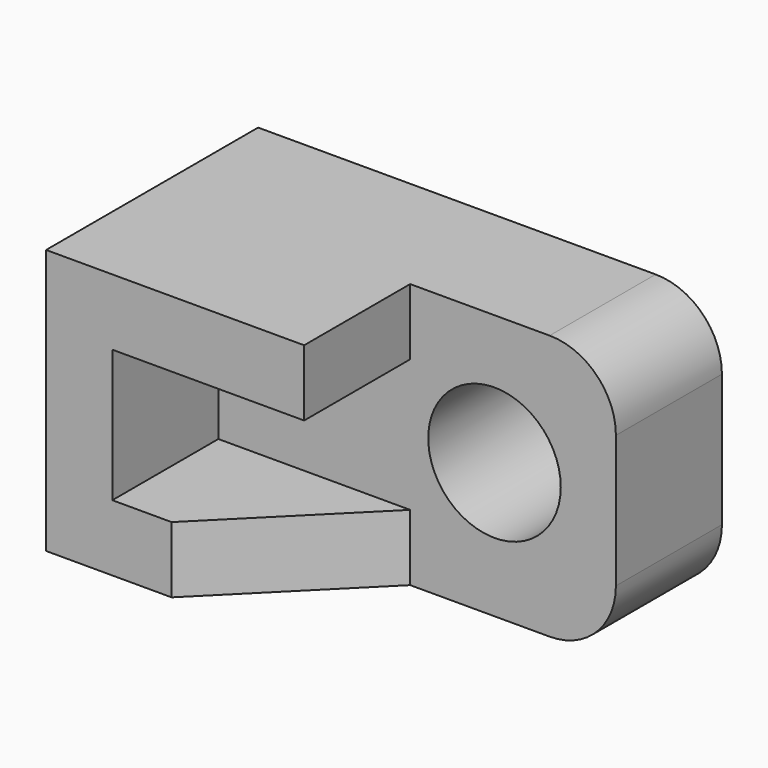
from build123d import *

# Parameters (mm, degrees)
F0_W      = 1778
F0_H      = 1016
F1_DEPTH  = 1016
F2_W      = 762
F2_H      = 508
F3_DEPTH  = 508
F4_W      = 26.7618985716
F4_H      = 508
F5_DEPTH  = 508
F6_R      = 254
F7_R      = 254
F8_R      = 254
F9_DEPTH  = 508
F11_DEPTH = 254


with BuildPart() as f1:
    # F0 (on Top) → F1 (new body)
    with BuildSketch(Plane.XY):
        with Locations((133.4459019247, 5.0370320678)):
            Rectangle(F0_W, F0_H)
    extrude(amount=F1_DEPTH)

    # F2 (on face) → F3 (cut)
    with BuildSketch(Plane.XZ.offset(502.9629679322)):
        with Locations((-120.5540980753, 508)):
            Rectangle(F2_W, F2_H)
    extrude(amount=-F3_DEPTH, mode=Mode.SUBTRACT)

    # F4 (on face) → F5 (cut)
    with BuildSketch(Plane.XZ.offset(502.9629679322)):
        with Locations((247.0649526389, 508)):
            Rectangle(F4_W, F4_H)
        Polygon((1022.4459019247, 1016), (233.6840033531, 1016), (233.6840033531, 762), (260.4459019247, 762), (260.4459019247, 254), (233.6840033531, 254), (233.6840033531, 0), (1022.4459019247, 0), align=None)
    extrude(amount=-F5_DEPTH, mode=Mode.SUBTRACT)

    # F6
    f6_edges = [f1.edges().sort_by_distance(p)[0] for p in [
        (1022.445902, 259.037032, 1016),
    ]]
    fillet(f6_edges, radius=F6_R)

    # F7
    f7_edges = [f1.edges().sort_by_distance(p)[0] for p in [
        (1022.445902, 259.037032, 0),
    ]]
    fillet(f7_edges, radius=F7_R)

    # F8 (on face) → F9 (cut)
    with BuildSketch(Plane.XZ.offset(-5.0370320678)):
        with Locations((557.0327043533, 518.402338028)):
            Circle(F8_R)
    extrude(amount=-F9_DEPTH, mode=Mode.SUBTRACT)

    # F10 (on face) → F11 (cut)
    with BuildSketch(Plane(origin=(0, 0, 0), x_dir=(1, 0, 0), z_dir=(0, 0, -1))):
        Polygon((233.6840033531, -5.0370320678), (233.6840033531, 502.9629679322), (-274.3159966469, 502.9629679322), align=None)
    extrude(amount=-F11_DEPTH, mode=Mode.SUBTRACT)


solid = f1.part
